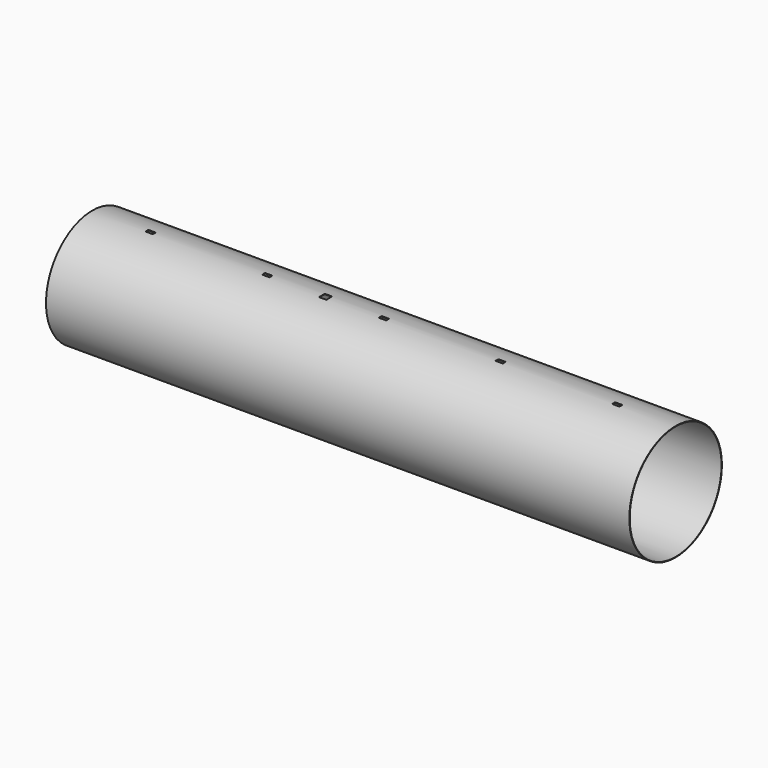
from build123d import *

# Parameters (mm, degrees)
F0_R          = 201.6125
F0_R_2        = 200.025
F1_DEPTH      = 2032
F2_W          = 25.4
F2_H          = 25.4
F3_DEPTH      = 508
F4_DEPTH      = 2714
F4_DEPTH_BACK = 709.6135
F5_W          = 25.4
F5_H          = 12.7
F6_DEPTH      = 201.6135
F6_DEPTH_BACK = 201.6135


# Not quite as in the source:
# - an extrude ends at something that could not be found from the text; its depth is read off the source's solid


with BuildPart() as f1:
    # F0 (on Right) → F1 (new body)
    with BuildSketch(Plane.YZ):
        Circle(F0_R)
        Circle(F0_R_2, mode=Mode.SUBTRACT)
    extrude(amount=F1_DEPTH)


with BuildPart() as f3:
    # F2 (on Top) → F3 (new body)
    with BuildSketch(Plane.XY):
        with Locations((812.8, 0)):
            Rectangle(F2_W, F2_H)
    extrude(amount=F3_DEPTH)


with BuildPart() as f4_tool:
    # F4 (cut, two sides): a face of the model
    f4_faces = [f3.part.faces().sort_by_distance(p)[0] for p in [
        (812.8, 0, 508),
    ]]
    extrude(f4_faces, amount=F4_DEPTH)
    extrude(f4_faces, amount=-F4_DEPTH_BACK)


with BuildPart() as f1_1:
    add(f1.part)

    # F4: cut by f4_tool
    add(f4_tool.part, mode=Mode.SUBTRACT)

    # F5 (on Top) → F6 (cut, two sides)
    with BuildSketch(Plane.XY) as f6_sk:
        with Locations((203.2, 0)):
            Rectangle(F5_W, F5_H)
        with Locations((609.6, 0)):
            Rectangle(F5_W, F5_H)
        with Locations((1016, 0)):
            Rectangle(F5_W, F5_H)
        with Locations((1422.4, 0)):
            Rectangle(F5_W, F5_H)
        with Locations((1828.8, 0)):
            Rectangle(F5_W, F5_H)
    extrude(amount=F6_DEPTH, mode=Mode.SUBTRACT)
    extrude(f6_sk.sketch, amount=-F6_DEPTH_BACK, mode=Mode.SUBTRACT)


with BuildPart() as f3_1:
    add(f3.part)

    # F4: cut by f4_tool
    add(f4_tool.part, mode=Mode.SUBTRACT)


solid = f1_1.part
